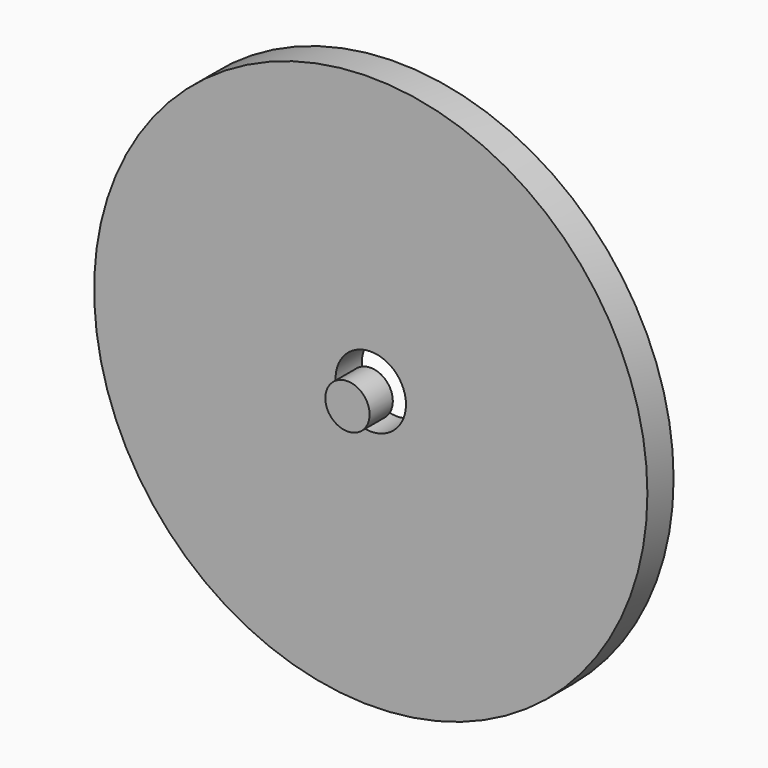
from build123d import *

# Parameters (mm, degrees)
F0_R     = 75.10308026
F0_R_2   = 9.559954458
F4_DEPTH = 8.89
F6_R     = 6.0103256088
F7_DEPTH = 7.874


# Not quite as in the source:
# - the program builds the solid bodies; features that only make, move or delete a surface that nothing else refers to are left out


with BuildPart() as f4:
    # F0 (on Front) → F4 (new body)
    with BuildSketch(Plane.XZ):
        Circle(F0_R)
        Circle(F0_R_2, mode=Mode.SUBTRACT)
    extrude(amount=-F4_DEPTH)


with BuildPart() as f7:
    # F6 (on Front) → F7 (new body)
    with BuildSketch(Plane.XZ):
        with Locations((-0.0235913109, -0.3345536048)):
            Circle(F6_R)
    extrude(amount=F7_DEPTH)


solid = Compound([f4.part, f7.part])
